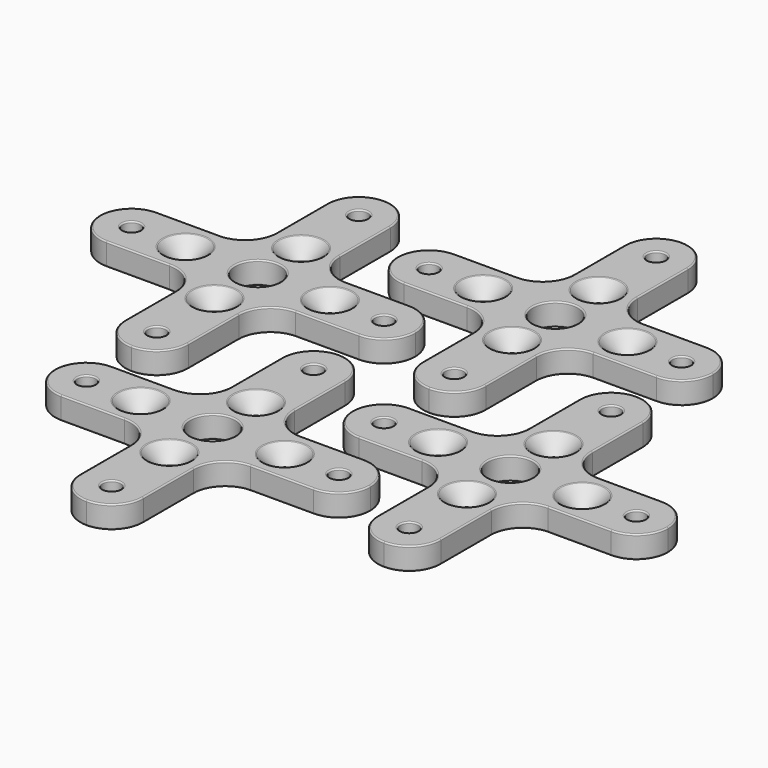
from build123d import *

# Parameters (mm, degrees)
F0_R     = 1
F0_R_2   = 0.8
F0_R_3   = 2.5
F1_DEPTH = 2.5
F2_R     = 3.49999
F3_SIZE  = 1.7
F4_R     = 0.15


# Not quite as in the source:
# - a fillet or chamfer is up to 0.001 mm smaller than in the source, because OpenCascade refuses the exact size


with BuildPart() as f1:
    # F0 (on Top) → F1 (new body)
    with BuildSketch(Plane.XY):
        Polygon((-24.8403990492, -37.8702705037), (-17.8403990492, -37.8702705037), (-17.8403990492, -23.8702705037), (-3.8403990492, -23.8702705037), (-3.8403990492, -16.8702705037), (-17.8403990492, -16.8702705037), (-17.8403990492, -2.8702705037), (-24.8403990492, -2.8702705037), (-24.8403990492, -16.8702705037), (-38.8403990492, -16.8702705037), (-38.8403990492, -23.8702705037), (-24.8403990492, -23.8702705037), align=None)
        with Locations((-21.3403990492, -34.3702705037)):
            Circle(F0_R, mode=Mode.SUBTRACT)
        with Locations((-21.3403990492, -26.3702705037)):
            Circle(F0_R_2, mode=Mode.SUBTRACT)
        with Locations((-35.3403990492, -20.3702705037)):
            Circle(F0_R, mode=Mode.SUBTRACT)
        with Locations((-29.3403990492, -20.3702705037)):
            Circle(F0_R_2, mode=Mode.SUBTRACT)
        with Locations((-21.3403990492, -14.3702705037)):
            Circle(F0_R_2, mode=Mode.SUBTRACT)
        with Locations((-21.3403990492, -6.3702705037)):
            Circle(F0_R, mode=Mode.SUBTRACT)
        with Locations((-21.3403990492, -20.3702705037)):
            Circle(F0_R_3, mode=Mode.SUBTRACT)
        with Locations((-13.3403990492, -20.3702705037)):
            Circle(F0_R_2, mode=Mode.SUBTRACT)
        with Locations((-7.3403990492, -20.3702705037)):
            Circle(F0_R, mode=Mode.SUBTRACT)
    extrude(amount=F1_DEPTH)

    # F2 (radius 3.5 in the source; OpenCascade refuses exactly that, so slightly less here)
    f2_edges = [f1.edges().sort_by_distance(p)[0] for p in [
        (-24.840399, -2.870271, 1.25),
        (-17.840399, -2.870271, 1.25),
        (-3.840399, -16.870271, 1.25),
        (-3.840399, -23.870271, 1.25),
        (-17.840399, -37.870271, 1.25),
        (-24.840399, -37.870271, 1.25),
        (-38.840399, -23.870271, 1.25),
        (-38.840399, -16.870271, 1.25),
        (-24.840399, -23.870271, 1.25),
        (-17.840399, -23.870271, 1.25),
        (-17.840399, -16.870271, 1.25),
        (-24.840399, -16.870271, 1.25),
    ]]
    fillet(f2_edges, radius=F2_R)

    # F3
    f3_edges = [f1.edges().sort_by_distance(p)[0] for p in [
        (-22.140399, -14.370271, 2.5),
        (-14.140399, -20.370271, 2.5),
        (-22.140399, -26.370271, 2.5),
        (-30.140399, -20.370271, 2.5),
    ]]
    chamfer(f3_edges, length=F3_SIZE)

    # F4
    f4_edges = [f1.edges().sort_by_distance(p)[0] for p in [
        (-23.840399, -14.370271, 2.5),
        (-31.840399, -23.870271, 2.5),
        (-37.815276, -22.845147, 2.5),
        (-25.865522, -24.895394, 2.5),
        (-38.840399, -20.370271, 2.5),
        (-24.840399, -30.870271, 2.5),
        (-37.815276, -17.895394, 2.5),
        (-23.815276, -36.845147, 2.5),
        (-31.840399, -16.870271, 2.5),
        (-21.340399, -37.870271, 2.5),
        (-25.865522, -15.845147, 2.5),
        (-18.865522, -36.845147, 2.5),
        (-24.840399, -9.870271, 2.5),
        (-17.840399, -30.870271, 2.5),
        (-23.815276, -3.895394, 2.5),
        (-16.815276, -24.895394, 2.5),
        (-21.340399, -2.870271, 2.5),
        (-10.840399, -23.870271, 2.5),
        (-18.865522, -3.895394, 2.5),
        (-4.865522, -22.845147, 2.5),
        (-17.840399, -9.870271, 2.5),
        (-3.840399, -20.370271, 2.5),
        (-16.815276, -15.845147, 2.5),
        (-4.865522, -17.895394, 2.5),
        (-10.840399, -16.870271, 2.5),
        (-22.340399, -34.370271, 2.5),
        (-36.340399, -20.370271, 2.5),
        (-22.340399, -6.370271, 2.5),
        (-23.840399, -20.370271, 2.5),
        (-8.340399, -20.370271, 2.5),
        (-15.840399, -20.370271, 2.5),
        (-23.840399, -26.370271, 2.5),
        (-31.840399, -20.370271, 2.5),
        (-31.840399, -23.870271, 0),
        (-37.815276, -22.845147, 0),
        (-25.865522, -24.895394, 0),
        (-38.840399, -20.370271, 0),
        (-24.840399, -30.870271, 0),
        (-37.815276, -17.895394, 0),
        (-23.815276, -36.845147, 0),
        (-31.840399, -16.870271, 0),
        (-21.340399, -37.870271, 0),
        (-25.865522, -15.845147, 0),
        (-18.865522, -36.845147, 0),
        (-24.840399, -9.870271, 0),
        (-17.840399, -30.870271, 0),
        (-23.815276, -3.895394, 0),
        (-16.815276, -24.895394, 0),
        (-21.340399, -2.870271, 0),
        (-10.840399, -23.870271, 0),
        (-18.865522, -3.895394, 0),
        (-4.865522, -22.845147, 0),
        (-17.840399, -9.870271, 0),
        (-3.840399, -20.370271, 0),
        (-16.815276, -15.845147, 0),
        (-4.865522, -17.895394, 0),
        (-10.840399, -16.870271, 0),
        (-22.340399, -34.370271, 0),
        (-22.140399, -26.370271, 0),
        (-36.340399, -20.370271, 0),
        (-30.140399, -20.370271, 0),
        (-22.140399, -14.370271, 0),
        (-22.340399, -6.370271, 0),
        (-23.840399, -20.370271, 0),
        (-14.140399, -20.370271, 0),
        (-8.340399, -20.370271, 0),
    ]]
    fillet(f4_edges, radius=F4_R)


with BuildPart() as f5_1:
    # F5: copy of F1
    add(f1.part.moved(Location((25, 10, 0))))


with BuildPart() as f6_1:
    # F6: copy of F1
    add(f1.part.moved(Location((15, -25, 0))))


with BuildPart() as f7_1:
    # F7: copy of F6_1
    add(f6_1.part.moved(Location((25, 10, 0))))


solid = Compound([f1.part, f5_1.part, f6_1.part, f7_1.part])
